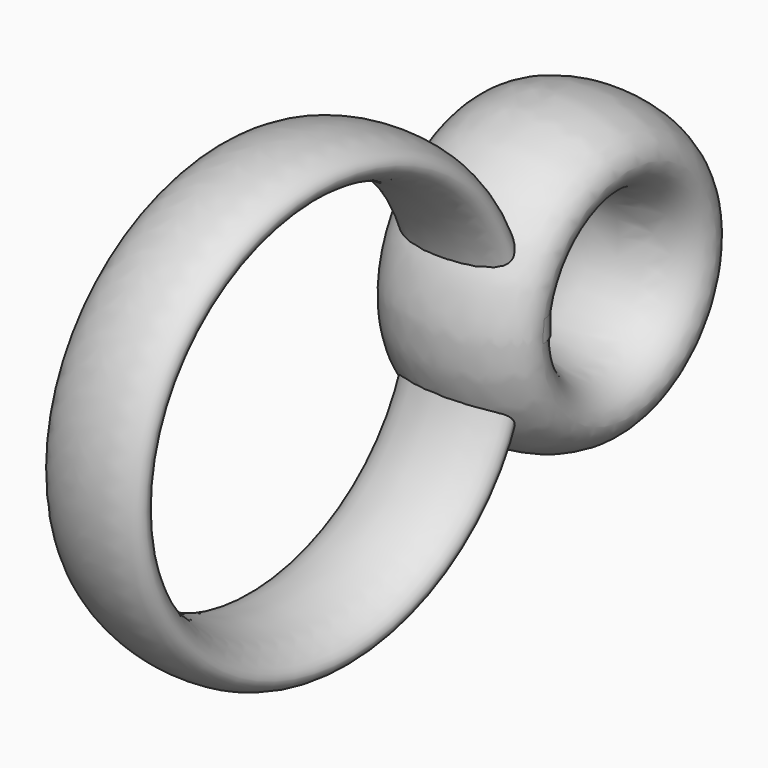
from build123d import *

# Parameters (mm, degrees)
F1_DEPTH = 25.4
F3_DEPTH = 25.4


with BuildPart() as f1:
    # F0 (on Top) → F1 (new body)
    with BuildSketch(Plane.XY):
        with BuildLine():
            add(Edge.make_bspline(
                [(95.1880961657, 0), (95.1880961657, 83.9109485248), (-47.5940480828, 41.9554742624), (-190.3761923313, 0), (-47.5940480828, -41.9554742624), (95.1880961657, -83.9109485248), (95.1880961657, 0)],
                knots=[0, 0, 0, 2.0943951024, 2.0943951024, 4.1887902048, 4.1887902048, 6.2831853072, 6.2831853072, 6.2831853072], degree=2, weights=[1, 0.5, 1, 0.5, 1, 0.5, 1]))
        make_face()
    extrude(amount=F1_DEPTH)


with BuildPart() as f3:
    # F2 (on face) → F3 (new body)
    with BuildSketch(Plane.XY.offset(25.4)):
        with BuildLine():
            add(Edge.make_bspline(
                [(68.1123584509, 0), (68.1123584509, 48.1318450904), (-34.0561792254, 24.0659225452), (-136.2247169018, 0), (-34.0561792254, -24.0659225452), (68.1123584509, -48.1318450904), (68.1123584509, 0)],
                knots=[0, 0, 0, 2.0943951024, 2.0943951024, 4.1887902048, 4.1887902048, 6.2831853072, 6.2831853072, 6.2831853072], degree=2, weights=[1, 0.5, 1, 0.5, 1, 0.5, 1]))
        make_face()
    extrude(amount=F3_DEPTH)


with BuildPart() as f5:
    # F1_face (on face) → F5 (revolve)
    with BuildSketch(Plane(origin=(0.5055157465, 0, 25.4), x_dir=(1, 0, 0), z_dir=(0, 0, 1))):
        with BuildLine():
            add(Edge.make_bspline(
                [(94.6825804191, 0), (94.6825804191, 83.9109485248), (-48.0995638294, 41.9554742624), (-190.8817080778, 0), (-48.0995638294, -41.9554742624), (94.6825804191, -83.9109485248), (94.6825804191, 0)],
                knots=[0, 0, 0, 2.0943951024, 2.0943951024, 4.1887902048, 4.1887902048, 6.2831853072, 6.2831853072, 6.2831853072], degree=2, weights=[1, 0.5, 1, 0.5, 1, 0.5, 1]))
        make_face()
    revolve(axis=Axis((12.4727413058, 127.1840631962, 0), (1, 0, 0)))


with BuildPart() as f7:
    # F3_face (on face) → F7 (revolve)
    with BuildSketch(Plane(origin=(0.361724534, 0, 50.8), x_dir=(1, 0, 0), z_dir=(0, 0, 1))):
        with BuildLine():
            add(Edge.make_bspline(
                [(67.7506339169, 0), (67.7506339169, 48.1318450904), (-34.4179037595, 24.0659225452), (-136.5864414358, 0), (-34.4179037595, -24.0659225452), (67.7506339169, -48.1318450904), (67.7506339169, 0)],
                knots=[0, 0, 0, 2.0943951024, 2.0943951024, 4.1887902048, 4.1887902048, 6.2831853072, 6.2831853072, 6.2831853072], degree=2, weights=[1, 0.5, 1, 0.5, 1, 0.5, 1]))
        make_face()
    revolve(axis=Axis((17.098814249, -246.9021379948, 0), (0.9956806191, -0.0928445197, 0)))


solid = Compound([f1.part, f3.part, f5.part, f7.part])
